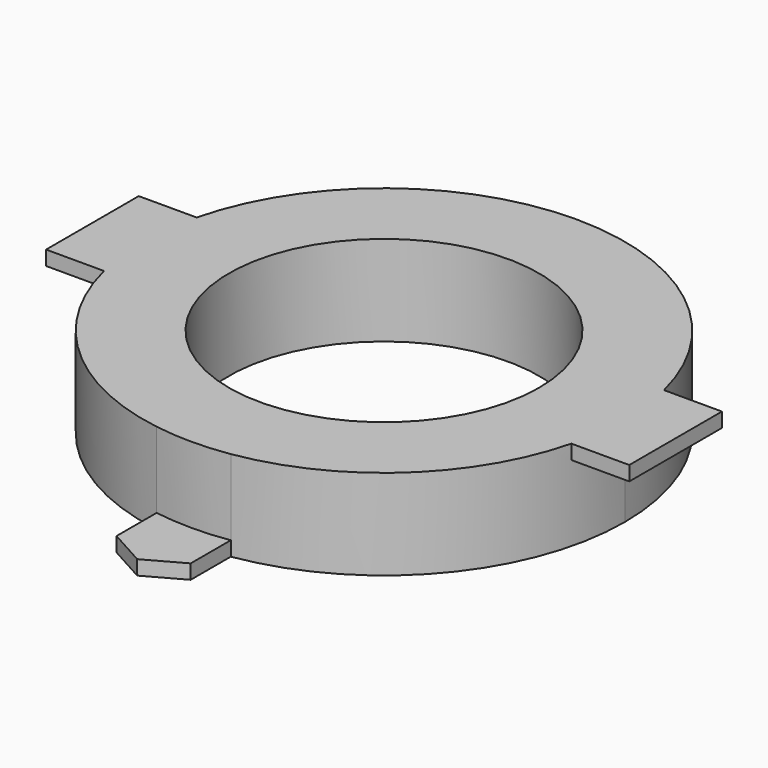
from build123d import *

# Parameters (mm, degrees)
F1_DEPTH = 6.24
F2_DEPTH = 1
F3_R     = 10.71
F4_DEPTH = 6.241
F6_DEPTH = 1


# Not quite as in the source:
# - a pattern or mirror of a feature is missing from the dataset's text; its kind, count and spacing are read off the source's solid


with BuildPart() as f1:
    # F0 (on Top) → F1 (new body)
    with BuildSketch(Plane.XY):
        with BuildLine():
            ThreePointArc((2.56, -16.4317771407), (12.6318981155, -10.8162863313), (16.63, 0))
            ThreePointArc((16.63, 0), (-10.8162863313, 12.6318981155), (-2.56, -16.4317771407))
            ThreePointArc((-2.56, -16.4317771407), (0, -16.63), (2.56, -16.4317771407))
        make_face()
    extrude(amount=F1_DEPTH)

    # F0 (on Top) → F2 (join)
    with BuildSketch(Plane.XY):
        with BuildLine():
            ThreePointArc((2.56, -16.4317771407), (0, -16.63), (-2.56, -16.4317771407))
            Line((-2.56, -16.4317771407), (-2.56, -19.8917771407))
            Line((-2.56, -19.8917771407), (0, -21.31))
            Line((0, -21.31), (2.56, -19.8917771407))
            Line((2.56, -19.8917771407), (2.56, -16.4317771407))
        make_face()
    extrude(amount=F2_DEPTH)

    # F3 (on face) → F4 (cut, through all)
    with BuildSketch(Plane.XY.offset(6.24)):
        Circle(F3_R)
    extrude(amount=-F4_DEPTH, mode=Mode.SUBTRACT)

    # F5 (on face) → F6 (join)
    with BuildSketch(Plane.XY.offset(6.24)):
        with BuildLine():
            Line((20.1417749953, 4), (16.1417749953, 4))
            ThreePointArc((16.1417749953, 4), (16.5074925136, 2.0148426524), (16.63, 0))
            ThreePointArc((16.63, 0), (16.5074925136, -2.0148426524), (16.1417749953, -4))
            Line((16.1417749953, -4), (20.1417749953, -4))
            Line((20.1417749953, -4), (20.1417749953, 4))
        make_face()
    f6 = extrude(amount=-F6_DEPTH)

    # F6_copies: F6 across plane
    add(f6.mirror(Plane(origin=(0, 0, 0), x_dir=(0, 0, -1), z_dir=(-1, 0, 0))))


solid = f1.part
